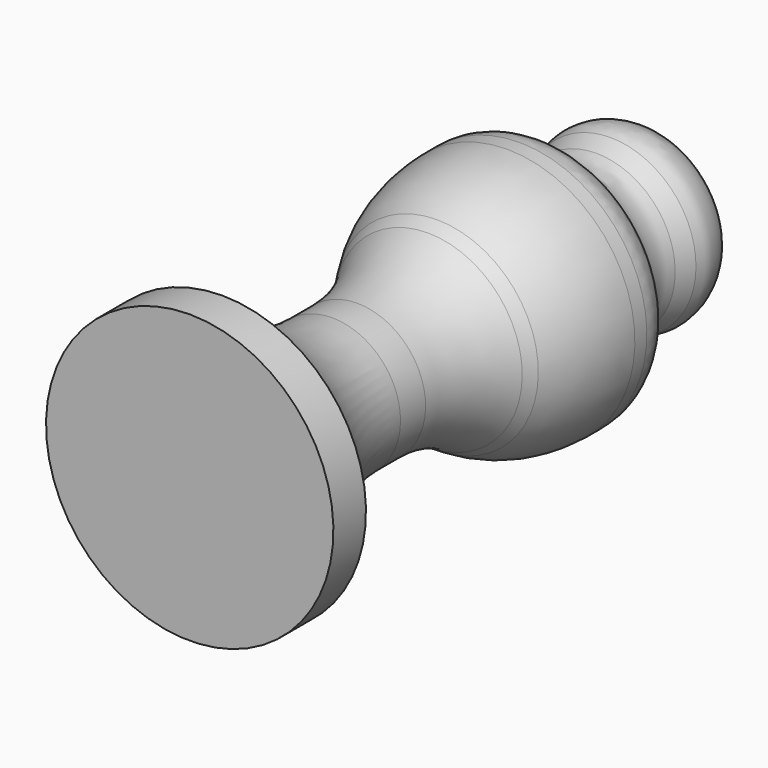
from build123d import *

# Parameters (mm, degrees)
F3_R = 1.27


# Not quite as in the source:
# - a fillet or chamfer that OpenCascade refuses, or shapes differently, is made with other operations: its cross-section is extruded or revolved along the edge and cut away or added


with BuildPart() as f1:
    # F0 (on Right) → F1 (revolve)
    with BuildSketch(Plane.YZ):
        Polygon((-19.05, 0), (0, 0), (0, 0.635), (-1.7329187831, 3.0259732157), (-4.0311289486, 2.1315128542), (-5.611469965, 3.9772258134), (-8.1580255717, 3.9772258134), (-11.0198768943, 2.1315128542), (-17.4555711955, 2.1315128542), (-17.78, 4.4826099296), (-19.05, 4.4826099296), align=None)
    revolve(axis=Axis((0, -9.525, 0), (0, -1, 0)))

    # F2: fillet of radius 5.08 on 3 edges, made by hand

    # F2_s1 → F2_t2 (revolve)
    with BuildSketch(Plane.YZ):
        with BuildLine():
            ThreePointArc((-9.7626119553, 2.94236916), (-11.0808174663, 2.3384414426), (-12.5159394181, 2.1315128542))
            Line((-12.5159394181, 2.1315128542), (-11.0198768943, 2.1315128542))
            Line((-11.0198768943, 2.1315128542), (-9.7626119553, 2.94236916))
        make_face()
    revolve(axis=Axis((0, -11.0198768943, 0), (0, -1, 0)))

    # F2_s3 → F2_t4 (revolve, cut)
    with BuildSketch(Plane.YZ):
        with BuildLine():
            ThreePointArc((-9.4152905107, 3.1663695077), (-8.0970849997, 3.7702972251), (-6.6619630479, 3.9772258134))
            Line((-6.6619630479, 3.9772258134), (-8.1580255717, 3.9772258134))
            Line((-8.1580255717, 3.9772258134), (-9.4152905107, 3.1663695077))
        make_face()
    revolve(axis=Axis((0, -8.1580255717, 0), (0, -1, 0)), mode=Mode.SUBTRACT)

    # F2_s5 → F2_t6 (revolve)
    with BuildSketch(Plane.YZ):
        with BuildLine():
            ThreePointArc((-17.78, 4.4826099296), (-15.9389265067, 2.7579060655), (-13.495202592, 2.1315128542))
            Line((-13.495202592, 2.1315128542), (-17.4555711955, 2.1315128542))
            Line((-17.4555711955, 2.1315128542), (-17.78, 4.4826099296))
        make_face()
    revolve(axis=Axis((0, -17.4555711955, 0), (0, -1, 0)))

    # F3
    f3_edges = [f1.edges().sort_by_distance(p)[0] for p in [
        (0, -5.61147, -3.977226),
        (0, -4.031129, -2.131513),
        (0, -1.732919, -3.025973),
    ]]
    fillet(f3_edges, radius=F3_R)


solid = f1.part
